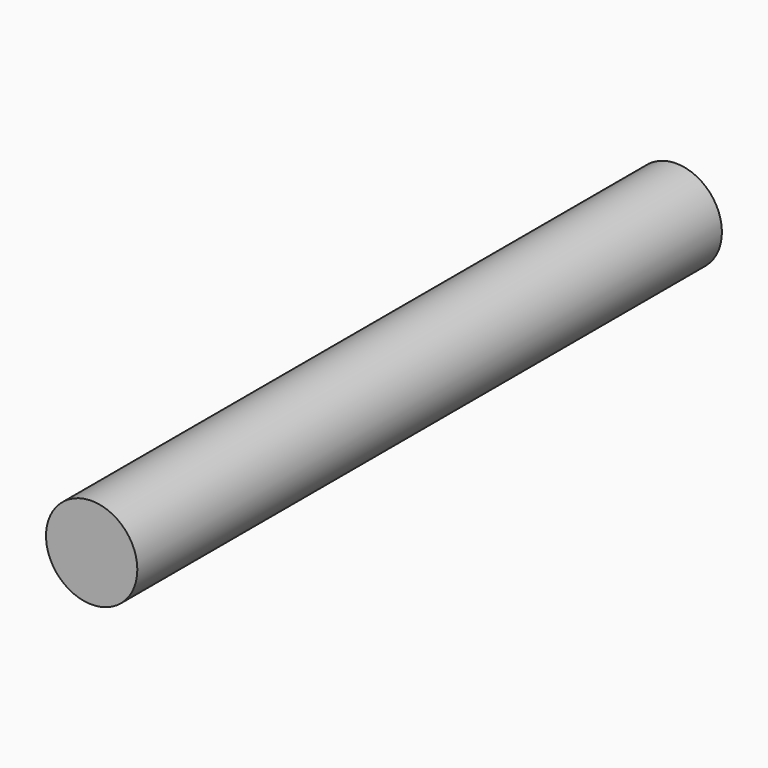
from build123d import *

# Parameters (mm, degrees)
F0_R     = 3.175
F1_DEPTH = 50.8


# Not quite as in the source:
# - a feature names something its author has since deleted; it is built from what else it names


with BuildPart() as f1:
    # F0 (on Front) → F1 (new body)
    with BuildSketch(Plane.XZ):
        Circle(F0_R)
    extrude(amount=F1_DEPTH)


solid = f1.part
